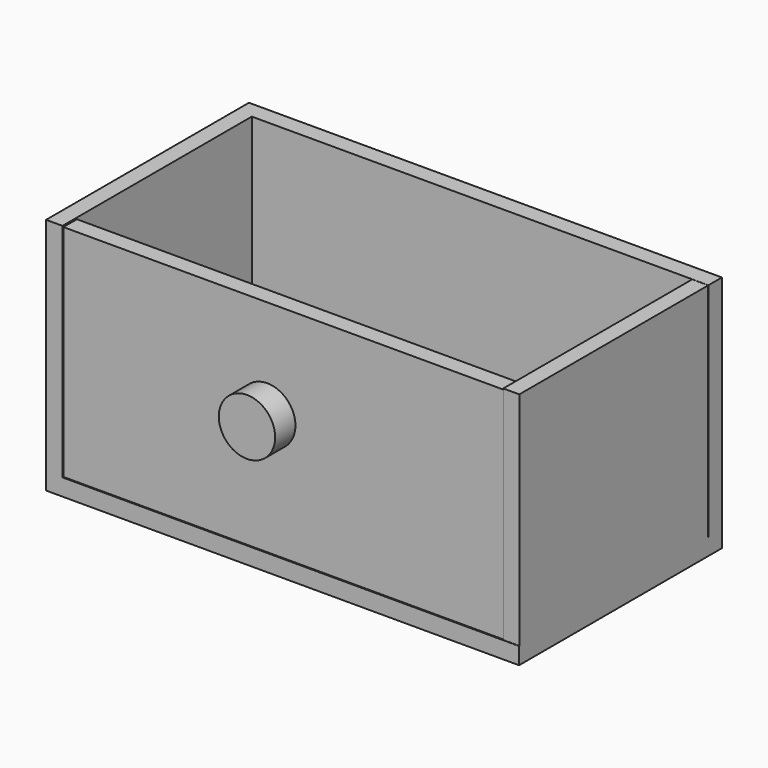
from build123d import *

# Parameters (mm, degrees)
F0_W      = 139.9
F0_H      = 75
F1_DEPTH  = 5
F2_W      = 139.9
F2_H      = 5
F5_DEPTH  = 65.5
F3_W      = 4.8456325173
F3_H      = 70
F6_DEPTH  = 65.5
F4_W      = 4.7526705265
F4_H      = 69.843
F7_DEPTH  = 65.5
F9_W      = 5
F9_H      = 65.0515219681
F10_DEPTH = 132.6
F11_R     = 8.3357715152
F12_DEPTH = 7.5


with BuildPart() as f1:
    # F0 (on Top) → F1 (new body)
    with BuildSketch(Plane.XY):
        with Locations((4.7975996614, -37.6802921295)):
            Rectangle(F0_W, F0_H)
    extrude(amount=F1_DEPTH)

    # F2 (on face) → F5 (join)
    with BuildSketch(Plane.XY.offset(5)):
        with Locations((4.7975996614, -2.6802921295)):
            Rectangle(F2_W, F2_H)
    extrude(amount=F5_DEPTH)

    # F3 (on face) → F6 (join)
    with BuildSketch(Plane.XY.offset(5)):
        with Locations((-62.72958408, -40.1802921295)):
            Rectangle(F3_W, F3_H)
    extrude(amount=F6_DEPTH)

    # F4 (on face) → F7 (join)
    with BuildSketch(Plane.XY.offset(5)):
        with Locations((72.3712643981, -40.1582837973)):
            Rectangle(F4_W, F4_H)
    extrude(amount=F7_DEPTH)

    # F9 (on face) → F10 (join)
    with BuildSketch(Plane.YZ.offset(-60.3067678213)):
        with Locations((-72.3428228498, 37.525760984)):
            Rectangle(F9_W, F9_H)
    extrude(amount=F10_DEPTH)

    # F11 (on face) → F12 (join)
    with BuildSketch(Plane.XZ.offset(74.8428228498)):
        with Locations((0, 40.6753867865)):
            Circle(F11_R)
    extrude(amount=F12_DEPTH)


solid = f1.part
